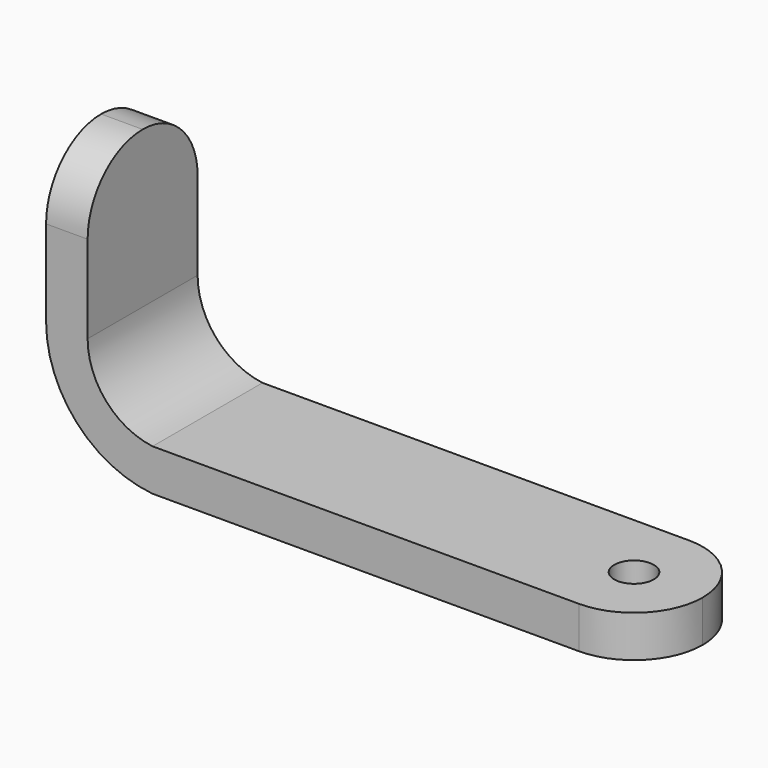
from build123d import *

# Parameters (mm, degrees)
F2_DEPTH = 4.8514
F3_R     = 4.85139
F4_R     = 1.397
F5_DEPTH = 25.4


# Not quite as in the source:
# - a variable given as a bare number and used for a length is read in inches; the dataset says mm whatever the document's units were
# - a fillet or chamfer is up to 0.001 mm smaller than in the source, because OpenCascade refuses the exact size


with BuildPart() as f2:
    # F1 (on Front) → F2 (new body, symmetric)
    with BuildSketch(Plane.XZ):
        with BuildLine():
            ThreePointArc((-7.5137404391, 8.2587754484), (-5.3542263452, 2.6761311983), (0, 0))
            Line((0, 0), (34.9550595609, 0))
            Line((34.9550595609, 0), (34.9550595609, 2.9464))
            Line((34.9550595609, 2.9464), (0, 2.9464))
            ThreePointArc((0, 2.9464), (-3.271499032, 4.6780426472), (-4.5800404391, 8.1405578545))
            Line((-4.5800404391, 8.1405578545), (-4.5800404391, 19.177))
            Line((-4.5800404391, 19.177), (-7.5137404391, 19.177))
            Line((-7.5137404391, 19.177), (-7.5137404391, 8.2587754484))
        make_face()
    extrude(amount=F2_DEPTH, both=True)

    # F3 (radius 4.8514 in the source; OpenCascade refuses exactly that, so slightly less here)
    f3_edges = [f2.edges().sort_by_distance(p)[0] for p in [
        (34.95506, -4.8514, 1.4732),
        (34.95506, 4.8514, 1.4732),
        (-6.04689, -4.8514, 19.177),
        (-6.04689, 4.8514, 19.177),
    ]]
    fillet(f3_edges, radius=F3_R)

    # F4 (on face) → F5 (cut)
    with BuildSketch(Plane.XY.offset(2.9464)):
        with Locations((30.1036595609, 0)):
            Circle(F4_R)
    extrude(amount=-F5_DEPTH, mode=Mode.SUBTRACT)


solid = f2.part
